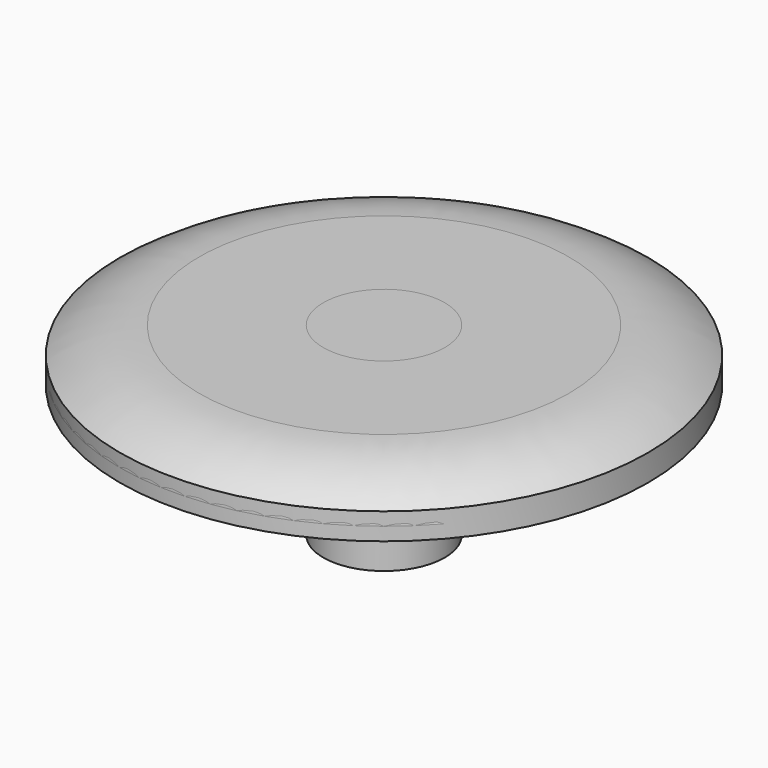
from build123d import *

# Parameters (mm, degrees)
F0_R     = 10
F0_R_2   = 2.3
F1_DEPTH = 1
F2_R     = 0.5
F3_DEPTH = 5
F4_DEPTH = 1
F5_DEPTH = 2
F6_DEPTH = 1
F7_SIZE  = 1


# Not quite as in the source:
# - a fillet or chamfer that OpenCascade refuses, or shapes differently, is made with other operations: its cross-section is extruded or revolved along the edge and cut away or added


with BuildPart() as f1:
    # F0 (on Top) → F1 (new body)
    with BuildSketch(Plane.XY):
        Circle(F0_R)
        Circle(F0_R_2, mode=Mode.SUBTRACT)
    extrude(amount=F1_DEPTH)

    # F2
    f2_edges = [f1.edges().sort_by_distance(p)[0] for p in [
        (-10, 0, 1),
    ]]
    fillet(f2_edges, radius=F2_R)

    # F0 (on Top) → F3 (join)
    with BuildSketch(Plane.XY):
        Circle(F0_R_2)
    extrude(amount=-F3_DEPTH)


with BuildPart() as f4:
    # F4 (new): a face of the model
    f4_faces = [f1.part.faces().sort_by_distance(p)[0] for p in [
        (0, 0, 0),
    ]]
    extrude(f4_faces, amount=F4_DEPTH)


with BuildPart() as f5:
    # F5 (new): a face of the model
    f5_faces = [f1.part.faces().sort_by_distance(p)[0] for p in [
        (-9.7171572875, 0, 0),
    ]]
    extrude(f5_faces, amount=-F5_DEPTH)

    # F7
    f7_edges = [f5.edges().sort_by_distance(p)[0] for p in [
        (-10, 0, 2),
    ]]
    chamfer(f7_edges, length=F7_SIZE)

    # F8: fillet of radius 5 on 1 edges, made by hand

    # F8_s1 → F8_t2 (revolve, cut)
    with BuildSketch(Plane.XZ):
        with BuildLine():
            ThreePointArc((10, 1), (8.5811388301, 1.7434164903), (7, 2))
            Line((7, 2), (9, 2))
            Line((9, 2), (10, 1))
        make_face()
    revolve(axis=Axis((0, 0, 2), (0, 0, 1)), mode=Mode.SUBTRACT)


with BuildPart() as f6:
    # F6 (new): a face of the model
    f6_faces = [f4.part.faces().sort_by_distance(p)[0] for p in [
        (0, 0, 1),
    ]]
    extrude(f6_faces, amount=F6_DEPTH)


solid = Compound([f1.part, f4.part, f5.part, f6.part])
